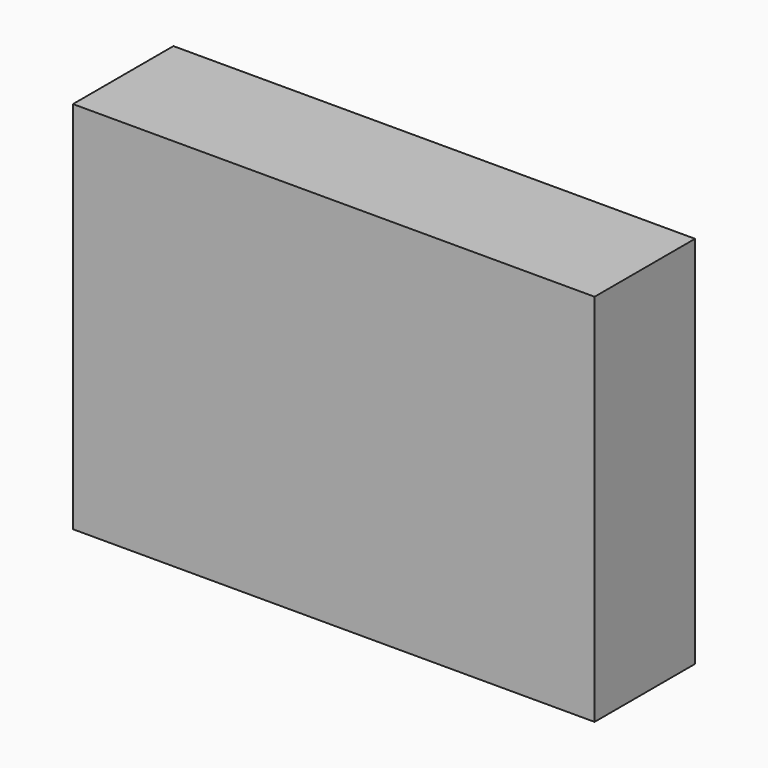
from build123d import *

# Parameters (mm, degrees)
F0_W     = 103.8585565984
F0_H     = 74.5262885466
F1_DEPTH = 25


# Not quite as in the source:
# - the program builds the solid bodies; features that only make, move or delete a surface that nothing else refers to are left out


with BuildPart() as f1:
    # F0 (on Front) → F1 (new body)
    with BuildSketch(Plane.XZ):
        with Locations((-16.8714690953, -23.0456213467)):
            Rectangle(F0_W, F0_H)
    extrude(amount=F1_DEPTH)


solid = f1.part
